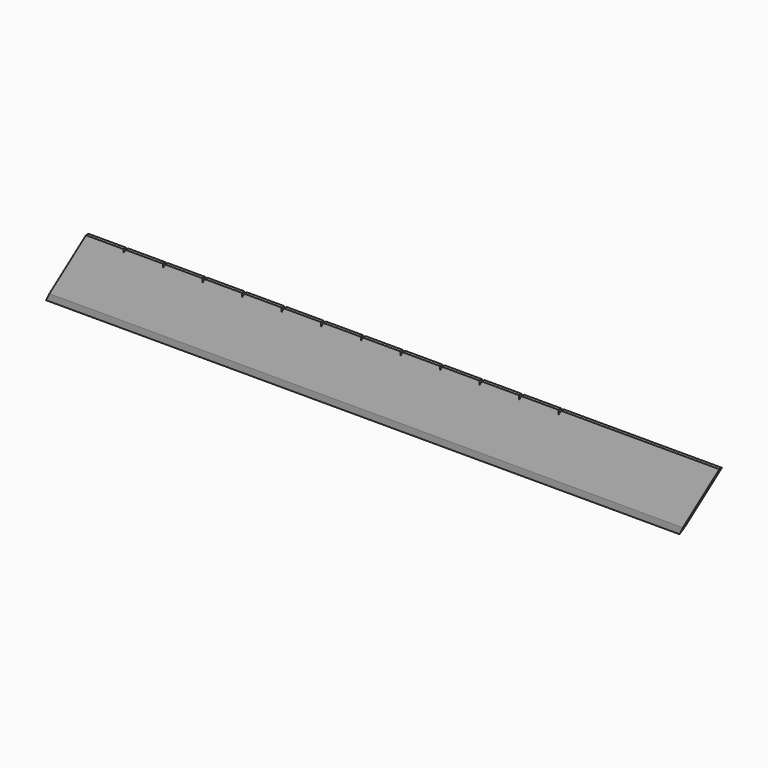
from build123d import *

# Parameters (mm, degrees)
F1_DEPTH   = 0.2
F2_SIZE2   = 0.2
F2_SIZE    = 1
F2_2_SIZE2 = 0.19999
F2_2_SIZE  = 0.99999


# Not quite as in the source:
# - a fillet or chamfer is up to 0.001 mm smaller than in the source, because OpenCascade refuses the exact size


with BuildPart() as f1:
    # F0 (on Front) → F1 (new body, symmetric)
    with BuildSketch(Plane.XZ):
        Polygon((5.1961524227, 9), (0, 0), (80, 0), (85.1961524227, 9), (65.1961524227, 9), (64.9074772881, 8.5), (64.9074772881, 9), (60.1961524227, 9), (59.9074772881, 8.5), (59.9074772881, 9), (55.1961524227, 9), (54.9074772881, 8.5), (54.9074772881, 9), (50.1961524227, 9), (49.9074772881, 8.5), (49.9074772881, 9), (45.1961524227, 9), (44.9074772881, 8.5), (44.9074772881, 9), (40.1961524227, 9), (39.9074772881, 8.5), (39.9074772881, 9), (35.1961524227, 9), (34.9074772881, 8.5), (34.9074772881, 9), (30.1961524227, 9), (29.9074772881, 8.5), (29.9074772881, 9), (25.1961524227, 9), (24.9074772881, 8.5), (24.9074772881, 9), (20.1961524227, 9), (19.9074772881, 8.5), (19.9074772881, 9), (15.1961524227, 9), (14.9074772881, 8.5), (14.9074772881, 9), (10.1961524227, 9), (9.9074772881, 8.5), (9.9074772881, 9), align=None)
    extrude(amount=F1_DEPTH, both=True)

    # F2
    f2_edges = [f1.edges().sort_by_distance(p)[0] for p in [
        (40, -0.2, 0),
    ]]
    f2_side = f1.faces().sort_by_distance((42.604211, -0.2, 4.494782))[0]
    chamfer(f2_edges, length=F2_SIZE, length2=F2_SIZE2, reference=f2_side)

    # F2#2 (size 1 and 0.2 in the source; OpenCascade refuses exactly that, so slightly less here)
    f2_2_edges = [f1.edges().sort_by_distance(p)[0] for p in [
        (40, 0.2, 0),
    ]]
    f2_2_side = f1.faces().sort_by_distance((42.604211, 0.2, 4.494782))[0]
    chamfer(f2_2_edges, length=F2_2_SIZE, length2=F2_2_SIZE2, reference=f2_2_side)


solid = f1.part
